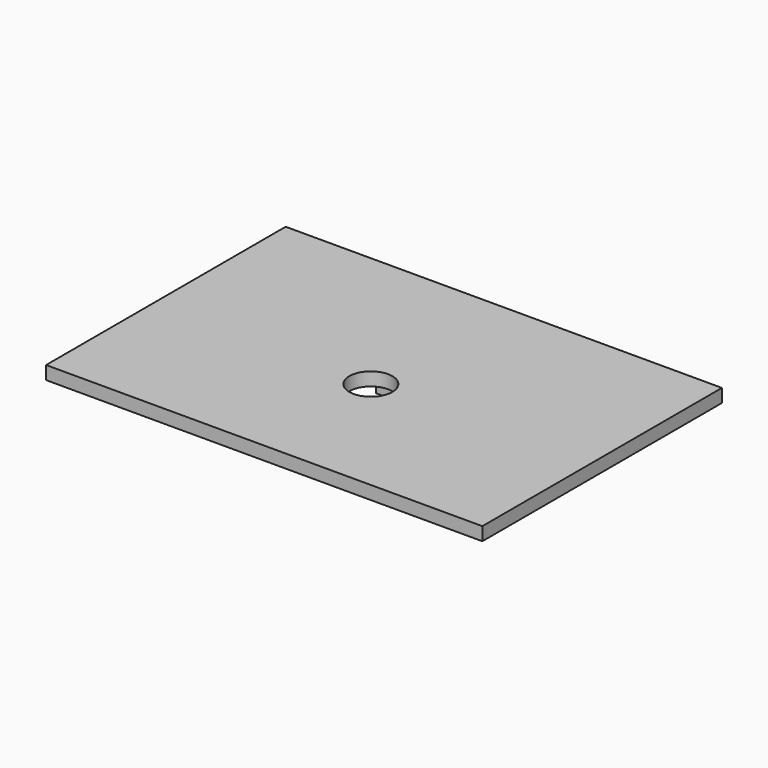
from build123d import *

# Parameters (mm, degrees)
F0_TEXT_SIZE = 9.7222222222
F1_DEPTH     = 1
F2_W         = 32.793527
F2_H         = 22.5120272536
F3_DEPTH     = 1
F5_R         = 1.6157504807
F6_DEPTH     = 1.001


# Not quite as in the source:
# - ends of sketch curves that miss each other by under 0.0002 mm in the source are joined
# - Text() gives the source's letters only with a copy of the font that has no kerning and outlines rounded to 1/6400 em; it was checked with that copy


with BuildPart() as f1:
    # F0 (on Top) → F1 (new body, symmetric)
    with BuildSketch(Plane.XY):
        with BuildLine():
            add(Edge.make_bspline(
                [(-3.127558, 3.9767104375), (-3.501983625, 4.0650346875), (-3.938088, 4.1089421875), (-4.436152875, 4.1089421875)],
                knots=[0, 0, 0, 0, 1, 1, 1, 1], degree=3))
            add(Edge.make_bspline(
                [(-4.436152875, 4.1089421875), (-4.948335, 4.1089133125), (-5.4537245, 4.0542144375), (-5.951780625, 3.9447388125)],
                knots=[0, 0, 0, 0, 1, 1, 1, 1], degree=3))
            add(Edge.make_bspline(
                [(-5.951780625, 3.9447388125), (-6.4498385, 3.8387684375), (-6.84334175, 3.7276880625), (-7.132986875, 3.6111223125)],
                knots=[0, 0, 0, 0, 1, 1, 1, 1], degree=3))
            Line((-7.132986875, 3.6111223125), (-7.132986875, 1.8993598125))
            Line((-7.132986875, 1.8993598125), (-6.93726075, 1.8993598125))
            add(Edge.make_bspline(
                [(-6.93726075, 1.8993598125), (-6.573431375, 2.1148294375), (-6.19717525, 2.2792708125), (-5.808625375, 2.3923085625)],
                knots=[0, 0, 0, 0, 1, 1, 1, 1], degree=3))
            add(Edge.make_bspline(
                [(-5.808625375, 2.3923085625), (-5.420067625, 2.5088576875), (-5.0597435, 2.5669988125), (-4.727708125, 2.5669988125)],
                knots=[0, 0, 0, 0, 1, 1, 1, 1], degree=3))
            add(Edge.make_bspline(
                [(-4.727708125, 2.5669988125), (-4.5934805, 2.5669988125), (-4.432490125, 2.5566738125), (-4.24527775, 2.5354629375)],
                knots=[0, 0, 0, 0, 1, 1, 1, 1], degree=3))
            add(Edge.make_bspline(
                [(-4.24527775, 2.5354629375), (-4.058065375, 2.5142564375), (-3.9530575, 2.4990760625), (-3.757996375, 2.4173878125)],
                knots=[0, 0, 0, 0, 1, 1, 1, 1], degree=3))
            add(Edge.make_bspline(
                [(-3.757996375, 2.4173878125), (-3.632603625, 2.3648790625), (-3.5057785, 2.3115731875), (-3.415083875, 2.2212618125)],
                knots=[0, 0, 0, 0, 1, 1, 1, 1], degree=3))
            add(Edge.make_bspline(
                [(-3.415083875, 2.2212618125), (-3.308816, 2.1154568125), (-3.21405175, 2.0251673125), (-3.212486375, 1.7934209375)],
                knots=[0, 0, 0, 0, 1, 1, 1, 1], degree=3))
            add(Edge.make_bspline(
                [(-3.212486375, 1.7934209375), (-3.21091225, 1.4841346875), (-3.25122175, 1.4139176875), (-3.32894275, 1.3008799375)],
                knots=[0, 0, 0, 0, 1, 1, 1, 1], degree=3))
            add(Edge.make_bspline(
                [(-3.32894275, 1.3008799375), (-3.406648, 1.1913824375), (-3.52331525, 1.1031518125), (-3.678733625, 1.0360086875)],
                knots=[0, 0, 0, 0, 1, 1, 1, 1], degree=3))
            add(Edge.make_bspline(
                [(-3.678733625, 1.0360086875), (-3.827093375, 0.9724688125), (-4.12351625, 0.9315748125), (-4.335457, 0.9138893125)],
                knots=[0, 0, 0, 0, 1, 1, 1, 1], degree=3))
            add(Edge.make_bspline(
                [(-4.335457, 0.9138893125), (-4.547396875, 0.8962020625), (-4.791061625, 0.8875946875), (-5.0665825, 0.8875946875)],
                knots=[0, 0, 0, 0, 1, 1, 1, 1], degree=3))
            Line((-5.0665825, 0.8875946875), (-5.517070125, 0.8875946875))
            Line((-5.517070125, 0.8875946875), (-5.517070125, -0.5216785625))
            Line((-5.517070125, -0.5216785625), (-5.08275775, -0.5216785625))
            add(Edge.make_bspline(
                [(-5.08275775, -0.5216785625), (-4.874354625, -0.5216785625), (-4.648343875, -0.5255915625), (-4.404609125, -0.5325600625)],
                knots=[0, 0, 0, 0, 1, 1, 1, 1], degree=3))
            add(Edge.make_bspline(
                [(-4.404609125, -0.5325600625), (-4.16088225, -0.5364721875), (-3.95211075, -0.5658161875), (-3.779022625, -0.6223298125)],
                knots=[0, 0, 0, 0, 1, 1, 1, 1], degree=3))
            add(Edge.make_bspline(
                [(-3.779022625, -0.6223298125), (-3.6059345, -0.6753093125), (-3.466456875, -0.7656976875), (-3.3604865, -0.8928596875)],
                knots=[0, 0, 0, 0, 1, 1, 1, 1], degree=3))
            add(Edge.make_bspline(
                [(-3.3604865, -0.8928596875), (-3.254516125, -1.0164901875), (-3.201562, -1.1929978125), (-3.201562, -1.4226030625)],
                knots=[0, 0, 0, 0, 1, 1, 1, 1], degree=3))
            add(Edge.make_bspline(
                [(-3.201562, -1.4226030625), (-3.201562, -1.6592713125), (-3.240689375, -1.8409580625), (-3.318433125, -1.9681200625)],
                knots=[0, 0, 0, 0, 1, 1, 1, 1], degree=3))
            add(Edge.make_bspline(
                [(-3.318433125, -1.9681200625), (-3.396138375, -2.0917514375), (-3.5003325, -2.1980586875), (-3.6310225, -2.2863680625)],
                knots=[0, 0, 0, 0, 1, 1, 1, 1], degree=3))
            add(Edge.make_bspline(
                [(-3.6310225, -2.2863680625), (-3.797045, -2.3994031875), (-3.99982975, -2.4734868125), (-4.240019, -2.5087781875)],
                knots=[0, 0, 0, 0, 1, 1, 1, 1], degree=3))
            add(Edge.make_bspline(
                [(-4.240019, -2.5087781875), (-4.480217, -2.5405476875), (-4.702784625, -2.5565129375), (-4.907658875, -2.5565129375)],
                knots=[0, 0, 0, 0, 1, 1, 1, 1], degree=3))
            add(Edge.make_bspline(
                [(-4.907658875, -2.5565129375), (-5.257364, -2.5565129375), (-5.64436425, -2.4893706875), (-6.068244875, -2.3551290625)],
                knots=[0, 0, 0, 0, 1, 1, 1, 1], degree=3))
            add(Edge.make_bspline(
                [(-6.068244875, -2.3551290625), (-6.488596625, -2.2209014375), (-6.850634875, -2.0620460625), (-7.154413, -1.8783634375)],
                knots=[0, 0, 0, 0, 1, 1, 1, 1], degree=3))
            Line((-7.154413, -1.8783634375), (-7.361055625, -1.8783634375))
            Line((-7.361055625, -1.8783634375), (-7.361055625, -3.6107444375))
            add(Edge.make_bspline(
                [(-7.361055625, -3.6107444375), (-7.06788075, -3.7379064375), (-6.6881815, -3.8528368125), (-6.221910625, -3.9552783125)],
                knots=[0, 0, 0, 0, 1, 1, 1, 1], degree=3))
            add(Edge.make_bspline(
                [(-6.221910625, -3.9552783125), (-5.752110875, -4.0577583125), (-5.19031625, -4.1089431875), (-4.536840875, -4.1089431875)],
                knots=[0, 0, 0, 0, 1, 1, 1, 1], degree=3))
            add(Edge.make_bspline(
                [(-4.536840875, -4.1089431875), (-3.964599625, -4.1089431875), (-3.479000875, -4.0504100625), (-3.07984775, -3.9338451875)],
                knots=[0, 0, 0, 0, 1, 1, 1, 1], degree=3))
            add(Edge.make_bspline(
                [(-3.07984775, -3.9338451875), (-2.677164875, -3.8137418125), (-2.32758575, -3.6424054375), (-2.03087325, -3.4198710625)],
                knots=[0, 0, 0, 0, 1, 1, 1, 1], degree=3))
            add(Edge.make_bspline(
                [(-2.03087325, -3.4198710625), (-1.773177875, -3.2251056875), (-1.576098125, -2.9952921875), (-1.43279325, -2.7344450625)],
                knots=[0, 0, 0, 0, 1, 1, 1, 1], degree=3))
            Line((-1.43279325, -2.7344450625), (-1.43279325, -4.1081373125))
            Line((-1.43279325, -4.1081373125), (1.34896825, -4.1081373125))
            add(Edge.make_bspline(
                [(1.34896825, -4.1081373125), (1.977723125, -4.1081373125), (2.52145775, -4.0620458125), (2.98065425, -3.9702408125)],
                knots=[0, 0, 0, 0, 1, 1, 1, 1], degree=3))
            add(Edge.make_bspline(
                [(2.98065425, -3.9702408125), (3.4398595, -3.8784025625), (3.862159875, -3.7160883125), (4.247187, -3.4829576875)],
                knots=[0, 0, 0, 0, 1, 1, 1, 1], degree=3))
            add(Edge.make_bspline(
                [(4.247187, -3.4829576875), (4.759376125, -3.1721130625), (5.182991625, -2.7269786875), (5.51856375, -2.1476796875)],
                knots=[0, 0, 0, 0, 1, 1, 1, 1], degree=3))
            add(Edge.make_bspline(
                [(5.51856375, -2.1476796875), (5.854137625, -1.5648430625), (6.022022125, -0.7424095625), (6.022022125, -0.0076834375)],
                knots=[0, 0, 0, 0, 1, 1, 1, 1], degree=3))
            add(Edge.make_bspline(
                [(6.022022125, -0.0076834375), (6.022022125, 0.7552981875), (5.864896625, 1.5815956875), (5.550514375, 2.1432328125)],
                knots=[0, 0, 0, 0, 1, 1, 1, 1], degree=3))
            add(Edge.make_bspline(
                [(5.550514375, 2.1432328125), (5.239679375, 2.7084005625), (4.81219725, 3.1569868125), (4.268215, 3.4890213125)],
                knots=[0, 0, 0, 0, 1, 1, 1, 1], degree=3))
            add(Edge.make_bspline(
                [(4.268215, 3.4890213125), (3.95031175, 3.6868299375), (3.5581315, 3.8387973125), (3.09185975, 3.9447676875)],
                knots=[0, 0, 0, 0, 1, 1, 1, 1], degree=3))
            add(Edge.make_bspline(
                [(3.09185975, 3.9447676875), (2.625595875, 4.0542433125), (2.071111875, 4.1089421875), (1.428224, 4.1089421875)],
                knots=[0, 0, 0, 0, 1, 1, 1, 1], degree=3))
            Line((1.428224, 4.1089421875), (-1.43279325, 4.1089421875))
            Line((-1.43279325, 4.1089421875), (-1.43279325, 2.7485980625))
            add(Edge.make_bspline(
                [(-1.43279325, 2.7485980625), (-1.472233, 2.8430359375), (-1.51323725, 2.9309288125), (-1.553701625, 3.0017408125)],
                knots=[0, 0, 0, 0, 1, 1, 1, 1], degree=3))
            add(Edge.make_bspline(
                [(-1.553701625, 3.0017408125), (-1.69499575, 3.2490035625), (-1.9106605, 3.4590971875), (-2.200314375, 3.6321774375)],
                knots=[0, 0, 0, 0, 1, 1, 1, 1], degree=3))
            add(Edge.make_bspline(
                [(-2.200314375, 3.6321774375), (-2.44403425, 3.7770004375), (-2.753141125, 3.8919308125), (-3.127558, 3.9767104375)],
                knots=[0, 0, 0, 0, 1, 1, 1, 1], degree=3))
        make_face()
        with BuildLine():
            Line((-1.43279325, 1.0618894375), (-1.43279325, -0.5374556875))
            add(Edge.make_bspline(
                [(-1.43279325, -0.5374556875), (-1.510576375, -0.4320724375), (-1.59945625, -0.3342868125), (-1.702108625, -0.2462994375)],
                knots=[0, 0, 0, 0, 1, 1, 1, 1], degree=3))
            add(Edge.make_bspline(
                [(-1.702108625, -0.2462994375), (-1.868122375, -0.1050131875), (-2.051938875, 0.0026231875), (-2.25328425, 0.0768083125)],
                knots=[0, 0, 0, 0, 1, 1, 1, 1], degree=3))
            add(Edge.make_bspline(
                [(-2.25328425, 0.0768083125), (-2.45462175, 0.1509908125), (-2.645339375, 0.2004860625), (-2.825486125, 0.2252153125)],
                knots=[0, 0, 0, 0, 1, 1, 1, 1], degree=3))
            Line((-2.825486125, 0.2252153125), (-2.825486125, 0.2992411875))
            add(Edge.make_bspline(
                [(-2.825486125, 0.2992411875), (-2.645339375, 0.3239713125), (-2.45462175, 0.3735050625), (-2.25328425, 0.4476481875)],
                knots=[0, 0, 0, 0, 1, 1, 1, 1], degree=3))
            add(Edge.make_bspline(
                [(-2.25328425, 0.4476481875), (-2.051938875, 0.5218333125), (-1.868122375, 0.6294626875), (-1.702108625, 0.7707559375)],
                knots=[0, 0, 0, 0, 1, 1, 1, 1], degree=3))
            add(Edge.make_bspline(
                [(-1.702108625, 0.7707559375), (-1.59945625, 0.8587441875), (-1.510592125, 0.9565289375), (-1.43279325, 1.0618894375)],
                knots=[0, 0, 0, 0, 1, 1, 1, 1], degree=3))
        make_face(mode=Mode.SUBTRACT)
        with BuildLine():
            Line((0.601659625, 2.6357458125), (1.11563375, 2.6357458125))
            add(Edge.make_bspline(
                [(1.11563375, 2.6357458125), (1.5536395, 2.6357458125), (1.880393375, 2.6164153125), (2.095863, 2.5775259375)],
                knots=[0, 0, 0, 0, 1, 1, 1, 1], degree=3))
            add(Edge.make_bspline(
                [(2.095863, 2.5775259375), (2.314869375, 2.5422319375), (2.528806, 2.4733230625), (2.737216125, 2.3708815625)],
                knots=[0, 0, 0, 0, 1, 1, 1, 1], degree=3))
            add(Edge.make_bspline(
                [(2.737216125, 2.3708815625), (3.146966375, 2.1624714375), (3.445304625, 1.8727545625), (3.632517875, 1.5018656875)],
                knots=[0, 0, 0, 0, 1, 1, 1, 1], degree=3))
            add(Edge.make_bspline(
                [(3.632517875, 1.5018656875), (3.823259125, 1.1345074375), (3.918424125, 0.5273178125), (3.918424125, 0.0080700625)],
                knots=[0, 0, 0, 0, 1, 1, 1, 1], degree=3))
            add(Edge.make_bspline(
                [(3.918424125, 0.0080700625), (3.918424125, -0.5147144375), (3.831890125, -1.1180444375), (3.65880375, -1.4748108125)],
                knots=[0, 0, 0, 0, 1, 1, 1, 1], degree=3))
            add(Edge.make_bspline(
                [(3.65880375, -1.4748108125), (3.485724375, -1.8280448125), (3.214050875, -2.1104598125), (2.843164625, -2.3224005625)],
                knots=[0, 0, 0, 0, 1, 1, 1, 1], degree=3))
            add(Edge.make_bspline(
                [(2.843164625, -2.3224005625), (2.62769325, -2.4389663125), (2.4068485, -2.5203028125), (2.1807835, -2.5662368125)],
                knots=[0, 0, 0, 0, 1, 1, 1, 1], degree=3))
            add(Edge.make_bspline(
                [(2.1807835, -2.5662368125), (1.954710625, -2.6086489375), (1.59955775, -2.6297005625), (1.11563375, -2.6297005625)],
                knots=[0, 0, 0, 0, 1, 1, 1, 1], degree=3))
            Line((1.11563375, -2.6297005625), (0.601659625, -2.6297005625))
            Line((0.601659625, -2.6297005625), (0.601659625, 2.6357458125))
        make_face(mode=Mode.SUBTRACT)
        with BuildLine():
            add(Edge.make_bspline(
                [(14.3967635, -0.0078295625), (14.3967635, -0.7425556875), (14.228981375, -1.5649034375), (13.89340925, -2.1477400625)],
                knots=[0, 0, 0, 0, 1, 1, 1, 1], degree=3))
            add(Edge.make_bspline(
                [(13.925195375, 2.1431820625), (14.239577625, 1.5815423125), (14.3967635, 0.7551520625), (14.3967635, -0.0078295625)],
                knots=[0, 0, 0, 0, 1, 1, 1, 1], degree=3))
            add(Edge.make_bspline(
                [(12.642963375, 3.4889924375), (13.18694825, 3.1569570625), (13.61435775, 2.7083480625), (13.925195375, 2.1431820625)],
                knots=[0, 0, 0, 0, 1, 1, 1, 1], degree=3))
            add(Edge.make_bspline(
                [(11.466702625, 3.9446600625), (11.932974375, 3.8386896875), (12.325060125, 3.6868010625), (12.642963375, 3.4889924375)],
                knots=[0, 0, 0, 0, 1, 1, 1, 1], degree=3))
            add(Edge.make_bspline(
                [(9.802981125, 4.1089133125), (10.445869, 4.1089133125), (11.000441375, 4.0541356875), (11.466702625, 3.9446600625)],
                knots=[0, 0, 0, 0, 1, 1, 1, 1], degree=3))
            Line((9.802981125, 4.1089133125), (6.941809, 4.1089133125))
            Line((6.941809, 4.1089133125), (6.941809, -4.1081749375))
            Line((6.941809, -4.1081749375), (9.723508375, -4.1081749375))
            add(Edge.make_bspline(
                [(11.35543675, -3.9704096875), (10.8962385, -4.0622549375), (10.352262375, -4.1081749375), (9.723508375, -4.1081749375)],
                knots=[0, 0, 0, 0, 1, 1, 1, 1], degree=3))
            add(Edge.make_bspline(
                [(12.6217735, -3.4829550625), (12.2367525, -3.7160865625), (11.81464025, -3.8785714375), (11.35543675, -3.9704096875)],
                knots=[0, 0, 0, 0, 1, 1, 1, 1], degree=3))
            add(Edge.make_bspline(
                [(13.89340925, -2.1477400625), (13.557837125, -2.7270390625), (13.133962625, -3.1721104375), (12.6217735, -3.4829550625)],
                knots=[0, 0, 0, 0, 1, 1, 1, 1], degree=3))
        make_face()
        with BuildLine():
            add(Edge.make_bspline(
                [(12.293267, 0.0080516875), (12.293267, 0.5272994375), (12.197891125, 1.1346929375), (12.007149875, 1.5020511875)],
                knots=[0, 0, 0, 0, 1, 1, 1, 1], degree=3))
            add(Edge.make_bspline(
                [(12.033639625, -1.4747810625), (12.206726, -1.1180173125), (12.293267, -0.5146776875), (12.293267, 0.0080516875)],
                knots=[0, 0, 0, 0, 1, 1, 1, 1], degree=3))
            add(Edge.make_bspline(
                [(11.2176785, -2.3225440625), (11.588567375, -2.1106033125), (11.86056025, -1.8280141875), (12.033639625, -1.4747810625)],
                knots=[0, 0, 0, 0, 1, 1, 1, 1], degree=3))
            add(Edge.make_bspline(
                [(10.555369125, -2.5662709375), (10.781434125, -2.5203351875), (11.00220975, -2.4391168125), (11.2176785, -2.3225440625)],
                knots=[0, 0, 0, 0, 1, 1, 1, 1], degree=3))
            add(Edge.make_bspline(
                [(9.490376875, -2.6298904375), (9.974300875, -2.6298904375), (10.3292945, -2.6086839375), (10.555369125, -2.5662709375)],
                knots=[0, 0, 0, 0, 1, 1, 1, 1], degree=3))
            Line((9.490376875, -2.6298904375), (8.97641675, -2.6298904375))
            Line((8.97641675, -2.6298904375), (8.97641675, 2.6359453125))
            Line((8.97641675, 2.6359453125), (9.490376875, 2.6359453125))
            add(Edge.make_bspline(
                [(10.470590375, 2.5776484375), (10.255119, 2.6165395625), (9.928380875, 2.6359453125), (9.490376875, 2.6359453125)],
                knots=[0, 0, 0, 0, 1, 1, 1, 1], degree=3))
            add(Edge.make_bspline(
                [(11.111709875, 2.3710049375), (10.903297125, 2.4734455625), (10.68959675, 2.5423246875), (10.470590375, 2.5776484375)],
                knots=[0, 0, 0, 0, 1, 1, 1, 1], degree=3))
            add(Edge.make_bspline(
                [(12.007149875, 1.5020511875), (11.819936625, 1.8729470625), (11.5214575, 2.1625939375), (11.111709875, 2.3710049375)],
                knots=[0, 0, 0, 0, 1, 1, 1, 1], degree=3))
        make_face(mode=Mode.SUBTRACT)
        Polygon((-14.3967635, -4.1081749375), (-8.706201875, -4.1081749375), (-8.706201875, -2.5822081875), (-12.36214525, -2.5822081875), (-12.36214525, 4.1089133125), (-14.3967635, 4.1089133125), align=None)
        with Locations((-11.2595486111, -14.3074108161)):
            Text('2017', F0_TEXT_SIZE, font='Open Sans', font_style=FontStyle.BOLD, text_align=(TextAlign.LEFT, TextAlign.BOTTOM))
    extrude(amount=F1_DEPTH, both=True)


with BuildPart() as f3:
    # F2 (on Top) → F3 (new body)
    with BuildSketch(Plane.XY):
        with Locations((0, -5.1471003143)):
            Rectangle(F2_W, F2_H)
    extrude(amount=F3_DEPTH)

    # F4: union F1
    add(f1.part)

    # F5 (on face) → F6 (cut, through all)
    with BuildSketch(Plane(origin=(0, 0, 0), x_dir=(1, 0, 0), z_dir=(0, 0, -1))):
        with Locations((0, 6.3842367381)):
            Circle(F5_R)
    extrude(amount=-F6_DEPTH, mode=Mode.SUBTRACT)


solid = f3.part
